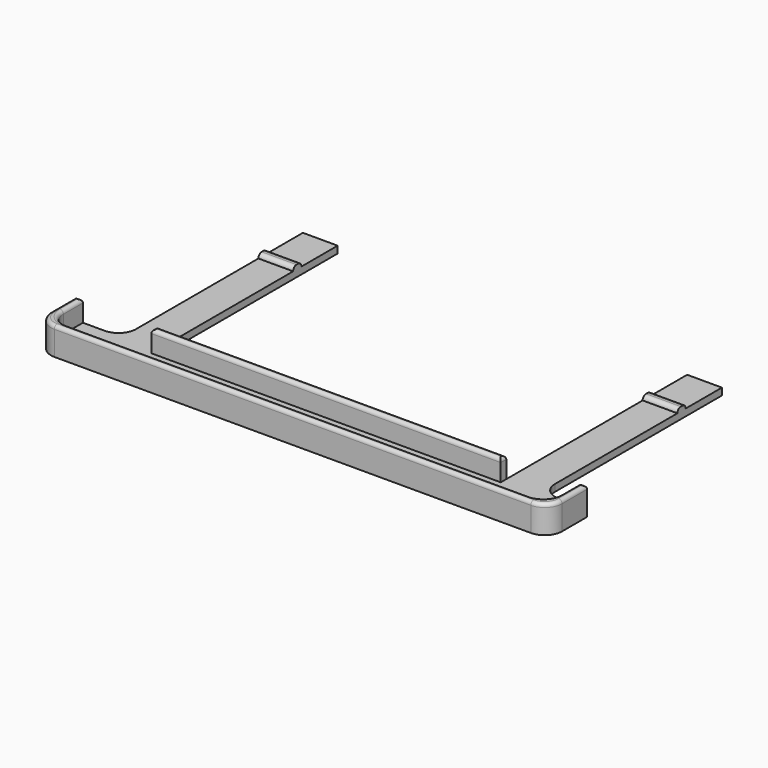
from build123d import *

# Parameters (mm, degrees)
F2_W     = 10
F2_H     = 65
F2_W_2   = 11.25
F2_H_2   = 12
F2_W_3   = 100.5
F2_H_3   = 2
F2_W_4   = 2
F2_H_4   = 10
F3_DEPTH = 2
F4_DEPTH = 8
F5_R     = 5
F6_R     = 0.99999
F7_W     = 10
F7_H     = 3
F8_DEPTH = 1.2
F9_R     = 1.19999


# Not quite as in the source:
# - a fillet or chamfer is up to 0.001 mm smaller than in the source, because OpenCascade refuses the exact size


with BuildPart() as f3:
    # F2 (on Top) → F3 (new body)
    with BuildSketch(Plane.XY):
        with Locations((-47.7500067828, 32.5)):
            Rectangle(F2_W, F2_H)
        Polygon((-42.7500067828, 0), (-52.7500067828, 0), (-52.7500067828, -12), (-42.7500067828, -12), (-42.7500067828, -2), align=None)
        with Locations((-58.3750067828, -6)):
            Rectangle(F2_W_2, F2_H_2)
        with Locations((7.4999932172, -1)):
            Rectangle(F2_W_3, F2_H_3)
        Polygon((-42.7500067828, -12), (-52.7500067828, -12), (-64.0000067828, -12), (-66.0000067828, -12), (-66.0000067828, -14), (80.9999932172, -14), (80.9999932172, -12), (78.9999932172, -12), (67.7499932172, -12), (57.7499932172, -12), align=None)
        with Locations((-65.0000067828, -6)):
            Rectangle(F2_W_4, F2_H_2)
        with Locations((62.7499932172, 32.5)):
            Rectangle(F2_W, F2_H)
        Polygon((67.7499932172, 0), (57.7499932172, 0), (57.7499932172, -2), (57.7499932172, -12), (67.7499932172, -12), align=None)
        with Locations((73.3749932172, -6)):
            Rectangle(F2_W_2, F2_H_2)
        with Locations((79.9999932172, -6)):
            Rectangle(F2_W_4, F2_H_2)
        with Locations((7.4999932172, -7)):
            Rectangle(F2_W_3, F2_H_4)
    extrude(amount=F3_DEPTH)

    # F2 (on Top) → F4 (join)
    with BuildSketch(Plane.XY):
        with Locations((-65.0000067828, -6)):
            Rectangle(F2_W_4, F2_H_2)
        Polygon((-42.7500067828, -12), (-52.7500067828, -12), (-64.0000067828, -12), (-66.0000067828, -12), (-66.0000067828, -14), (80.9999932172, -14), (80.9999932172, -12), (78.9999932172, -12), (67.7499932172, -12), (57.7499932172, -12), align=None)
        with Locations((79.9999932172, -6)):
            Rectangle(F2_W_4, F2_H_2)
        with Locations((7.4999932172, -1)):
            Rectangle(F2_W_3, F2_H_3)
    extrude(amount=F4_DEPTH)

    # F5
    f5_edges = [f3.edges().sort_by_distance(p)[0] for p in [
        (-66.000007, -14, 4),
        (80.999993, -14, 4),
        (-64.000007, -12, 5),
        (78.999993, -12, 5),
        (67.749993, 0, 1),
        (-52.750007, 0, 1),
    ]]
    fillet(f5_edges, radius=F5_R)

    # F6 (radius 1 in the source; OpenCascade refuses exactly that, so slightly less here)
    f6_edges = [f3.edges().sort_by_distance(p)[0] for p in [
        (7.499993, -14, 8),
        (7.499993, -12, 8),
        (79.999993, 0, 8),
        (-65.000007, 0, 8),
        (7.499993, -2, 8),
        (7.499993, 0, 8),
        (57.749993, -1, 8),
        (-42.750007, -1, 8),
    ]]
    fillet(f6_edges, radius=F6_R)

    # F7 (on face) → F8 (join)
    with BuildSketch(Plane.XY.offset(2)):
        with Locations((-47.7500067828, 50.5)):
            Rectangle(F7_W, F7_H)
        with Locations((62.7499932172, 50.5)):
            Rectangle(F7_W, F7_H)
    extrude(amount=F8_DEPTH)

    # F9 (radius 1.2 in the source; OpenCascade refuses exactly that, so slightly less here)
    f9_edges = [f3.edges().sort_by_distance(p)[0] for p in [
        (-47.750007, 49, 3.2),
        (-47.750007, 52, 3.2),
        (62.749993, 49, 3.2),
        (62.749993, 52, 3.2),
    ]]
    fillet(f9_edges, radius=F9_R)


solid = f3.part
